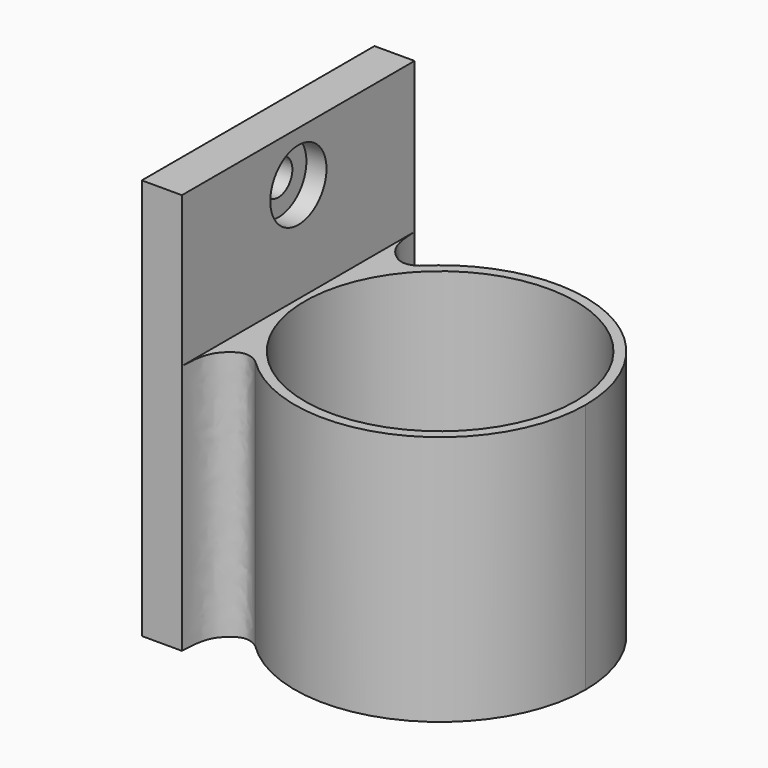
from build123d import *

# Parameters (mm, degrees)
F1_DEPTH = 40
F0_R     = 13.5
F2_DEPTH = 3
F3_DEPTH = 25
F4_R     = 1.75
F5_DEPTH = 25
F4_R_2   = 3.5
F6_DEPTH = 2


with BuildPart() as f1:
    # F0 (on Top) → F1 (new body)
    with BuildSketch(Plane.XY):
        with BuildLine():
            Line((-14.1355262175, -3.2306189119), (-14.1355262175, 3.2306189119))
            ThreePointArc((-14.1355262175, 3.2306189119), (-14.5, 0), (-14.1355262175, -3.2306189119))
        make_face()
        with BuildLine():
            ThreePointArc((-14.1355262175, -3.2306189119), (-14.5, 0), (-14.1355262175, 3.2306189119))
            Line((-14.1355262175, 3.2306189119), (-14.1355262175, 14.4821423069))
            Line((-14.1355262175, 14.4821423069), (-18.1355262175, 14.4821423069))
            Line((-18.1355262175, 14.4821423069), (-18.1355262175, -14.5178576931))
            Line((-18.1355262175, -14.5178576931), (-14.1355262175, -14.5178576931))
            Line((-14.1355262175, -14.5178576931), (-14.1355262175, -3.2306189119))
        make_face()
    extrude(amount=F1_DEPTH)

    # F0 (on Top) → F3 (join)
    with BuildSketch(Plane.XY):
        with BuildLine():
            ThreePointArc((-14.1355262175, 3.2306189119), (-12.6971385159, 7.0023334331), (-10.2746975407, 10.2313533048))
            add(Edge.make_bspline(
                [(-14.1355262175, 14.4821423069), (-14.0662710763, 12.0975714625), (-13.2319243302, 10.509407647), (-11.3992663412, 9.490766824), (-10.2746975407, 10.2313533048)],
                knots=[0, 0, 0, 0, 0.5620764572, 1, 1, 1, 1], degree=3))
            Line((-14.1355262175, 14.4821423069), (-14.1355262175, 3.2306189119))
        make_face()
        with BuildLine():
            ThreePointArc((-10.1697726735, -10.3356530403), (5.6030481095, -13.3737000072), (14.5, 0))
            ThreePointArc((14.5, 0), (5.5347486691, 13.402110176), (-10.2746975407, 10.2313533048))
            ThreePointArc((-10.2746975407, 10.2313533048), (-12.6971385159, 7.0023334331), (-14.1355262175, 3.2306189119))
            Line((-14.1355262175, 3.2306189119), (-14.1355262175, -3.2306189119))
            ThreePointArc((-14.1355262175, -3.2306189119), (-12.6612505716, -7.0670173314), (-10.1697726735, -10.3356530403))
        make_face()
        Circle(F0_R, mode=Mode.SUBTRACT)
        with BuildLine():
            add(Edge.make_bspline(
                [(-14.1355262175, -14.5178576931), (-14.1023624483, -11.961212262), (-13.2307772223, -10.5113467824), (-11.3579562474, -9.4215989986), (-10.1697726735, -10.3356530403)],
                knots=[0, 0, 0, 0, 0.5597409936, 1, 1, 1, 1], degree=3))
            ThreePointArc((-10.1697726735, -10.3356530403), (-12.6612505716, -7.0670173314), (-14.1355262175, -3.2306189119))
            Line((-14.1355262175, -3.2306189119), (-14.1355262175, -14.5178576931))
        make_face()
    extrude(amount=F3_DEPTH)

    # F4 (on face) → F5 (cut)
    with BuildSketch(Plane.YZ.offset(-14.1355262175)):
        with Locations((0, 35)):
            Circle(F4_R)
    extrude(amount=-F5_DEPTH, mode=Mode.SUBTRACT)

    # F4 (on face) → F6 (cut)
    with BuildSketch(Plane.YZ.offset(-14.1355262175)):
        with Locations((0, 35)):
            Circle(F4_R_2)
        with Locations((0, 35)):
            Circle(F4_R, mode=Mode.SUBTRACT)
    extrude(amount=-F6_DEPTH, mode=Mode.SUBTRACT)


with BuildPart() as f2:
    # F0 (on Top) → F2 (new body)
    with BuildSketch(Plane.XY):
        Circle(F0_R)
    extrude(amount=F2_DEPTH)


solid = Compound([f1.part, f2.part])
